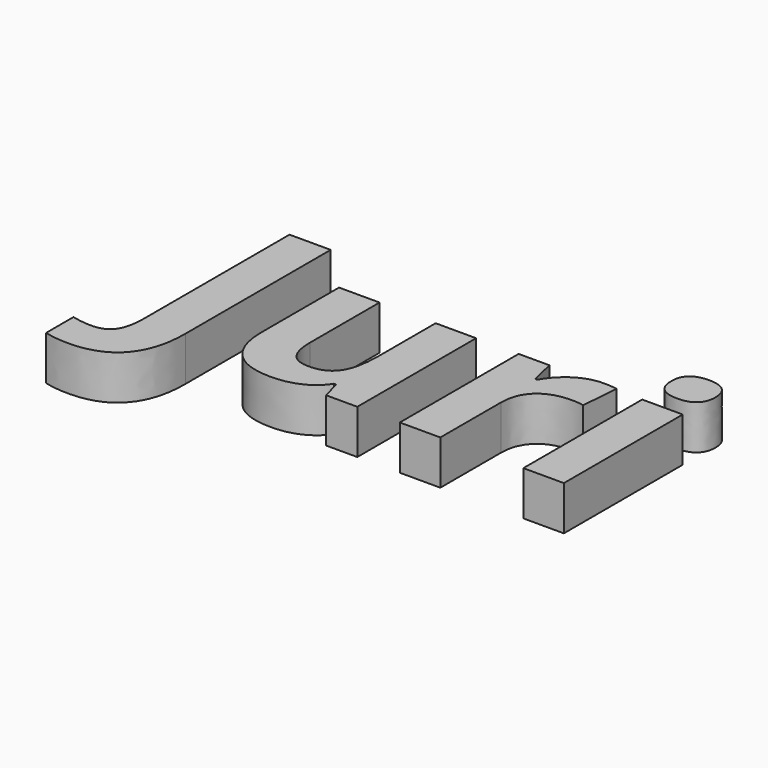
from build123d import *

# Parameters (mm, degrees)
F0_TEXT_SIZE = 156.1575776173
F1_DEPTH     = 25.4


# Not quite as in the source:
# - Text() gives the source's letters only with a copy of the font that has no kerning and outlines rounded to 1/6400 em; it was checked with that copy


with BuildPart() as f1:
    # F0 (on Top) → F1 (new body)
    with BuildSketch(Plane.XY):
        with Locations((-83.0056890845, -54.2225502431)):
            Text('Juri', F0_TEXT_SIZE, font='Open Sans', font_style=FontStyle.BOLD, text_align=(TextAlign.LEFT, TextAlign.BOTTOM))
    extrude(amount=F1_DEPTH)


solid = f1.part
